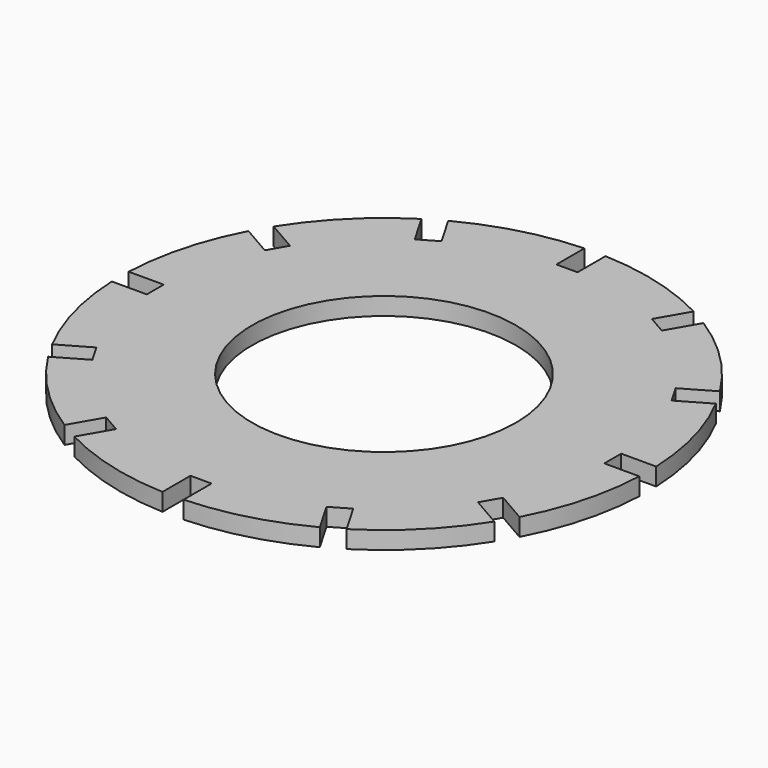
from build123d import *

# Parameters (mm, degrees)
F0_R            = 75
F0_R_2          = 37.5
F1_DEPTH        = 5
F3_DEPTH        = 52.7
F3_COPIES_COUNT = 12


# Not quite as in the source:
# - a pattern or mirror of a feature is missing from the dataset's text; its kind, count and spacing are read off the source's solid


with BuildPart() as f1:
    # F0 (on Top) → F1 (new body)
    with BuildSketch(Plane.XY):
        Circle(F0_R)
        Circle(F0_R_2, mode=Mode.SUBTRACT)
    extrude(amount=F1_DEPTH)

    # F2 (on face) → F3 (cut)
    with BuildSketch(Plane.XY.offset(5)):
        Polygon((3, -65), (-3, -65), (-3, -75), (0, -75), (3, -74.9399759808), align=None)
        Polygon((3, -74.9399759808), (0, -75), (3, -75), align=None)
    f3 = extrude(amount=-F3_DEPTH, mode=Mode.SUBTRACT)

    # F3_copies: F3 ×12 about axis
    f3_copies_axis = Axis((0, 0, 0), (0, 0, 1))
    for i in range(1, F3_COPIES_COUNT):
        add(f3.rotate(f3_copies_axis, i * 360 / F3_COPIES_COUNT), mode=Mode.SUBTRACT)


solid = f1.part
